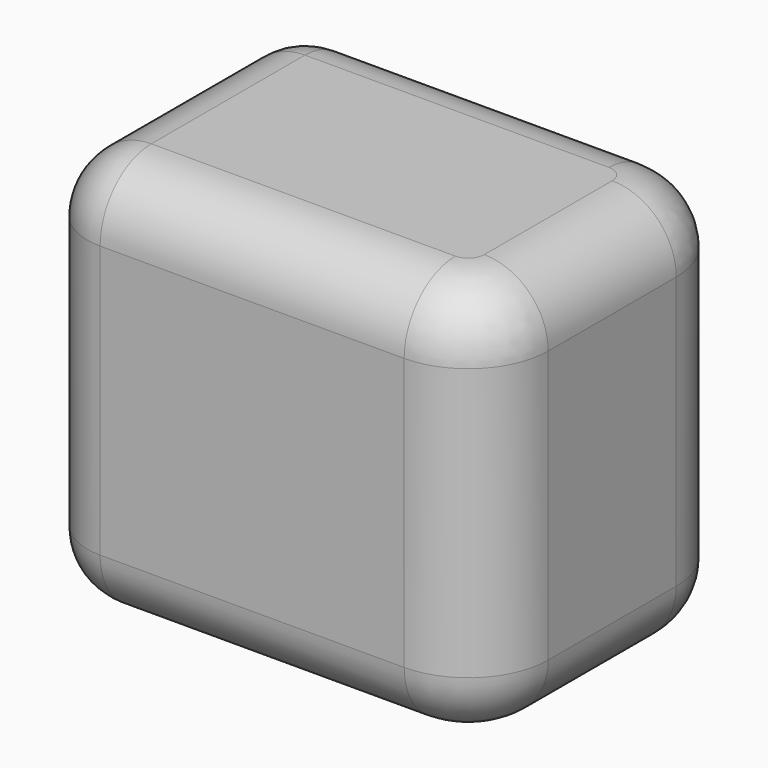
from build123d import *

# Parameters (mm, degrees)
F0_W        = 35.56
F0_H        = 31.75
F1_DEPTH    = 12.7
F2_R        = 5.08
F3_T1_DEPTH = 47.625
F3_T4_ANGLE = 90
F3_T6_ANGLE = 90
F4_R        = 5.08
F5_R        = 5.08


# Not quite as in the source:
# - a fillet or chamfer that OpenCascade refuses, or shapes differently, is made with other operations: its cross-section is extruded or revolved along the edge and cut away or added


with BuildPart() as f1:
    # F0 (on Front) → F1 (new body, symmetric)
    with BuildSketch(Plane.XZ):
        Rectangle(F0_W, F0_H)
    extrude(amount=F1_DEPTH, both=True)

    # F2
    f2_edges = [f1.edges().sort_by_distance(p)[0] for p in [
        (0, -12.7, 15.875),
        (0, 12.7, 15.875),
        (17.78, 0, 15.875),
    ]]
    fillet(f2_edges, radius=F2_R)

    # F3: fillet of radius 6.35 on 2 edges, made by hand

    # F3_s2 → F3_t1 (cut)
    with BuildSketch(Plane.XY.offset(-31.75)):
        with BuildLine():
            ThreePointArc((11.43, -12.7), (15.9201280605, -10.8401280605), (17.78, -6.35))
            Line((17.78, -6.35), (17.78, -12.7))
            Line((17.78, -12.7), (11.43, -12.7))
        make_face()
        with BuildLine():
            ThreePointArc((11.43, 12.7), (15.9201280605, 10.8401280605), (17.78, 6.35))
            Line((17.78, 6.35), (17.78, 12.7))
            Line((17.78, 12.7), (11.43, 12.7))
        make_face()
    extrude(amount=F3_T1_DEPTH, mode=Mode.SUBTRACT)

    # F3_s3 → F3_t4 (revolve, cut)
    with BuildSketch(Plane.XZ.offset(-6.35)):
        with BuildLine():
            ThreePointArc((12.7, 15.875), (16.2921024484, 14.3871024484), (17.78, 10.795))
            Line((17.78, 10.795), (17.78, 15.875))
            Line((17.78, 15.875), (12.7, 15.875))
        make_face()
    revolve(axis=Axis((11.43, 6.35, 15.875), (0, 0, 1)), revolution_arc=F3_T4_ANGLE, mode=Mode.SUBTRACT)

    # F3_s5 → F3_t6 (revolve, cut)
    with BuildSketch(Plane.YZ.offset(11.43)):
        with BuildLine():
            ThreePointArc((-7.62, 15.875), (-11.2121024484, 14.3871024484), (-12.7, 10.795))
            Line((-12.7, 10.795), (-12.7, 15.875))
            Line((-12.7, 15.875), (-7.62, 15.875))
        make_face()
    revolve(axis=Axis((11.43, -6.35, 15.875), (0, 0, 1)), revolution_arc=F3_T6_ANGLE, mode=Mode.SUBTRACT)

    # F4
    f4_edges = [f1.edges().sort_by_distance(p)[0] for p in [
        (-17.78, 0, -15.875),
    ]]
    fillet(f4_edges, radius=F4_R)

    # F5
    f5_edges = [f1.edges().sort_by_distance(p)[0] for p in [
        (-16.292102, -12.7, -14.387102),
        (-16.292102, 12.7, -14.387102),
    ]]
    fillet(f5_edges, radius=F5_R)


solid = f1.part
